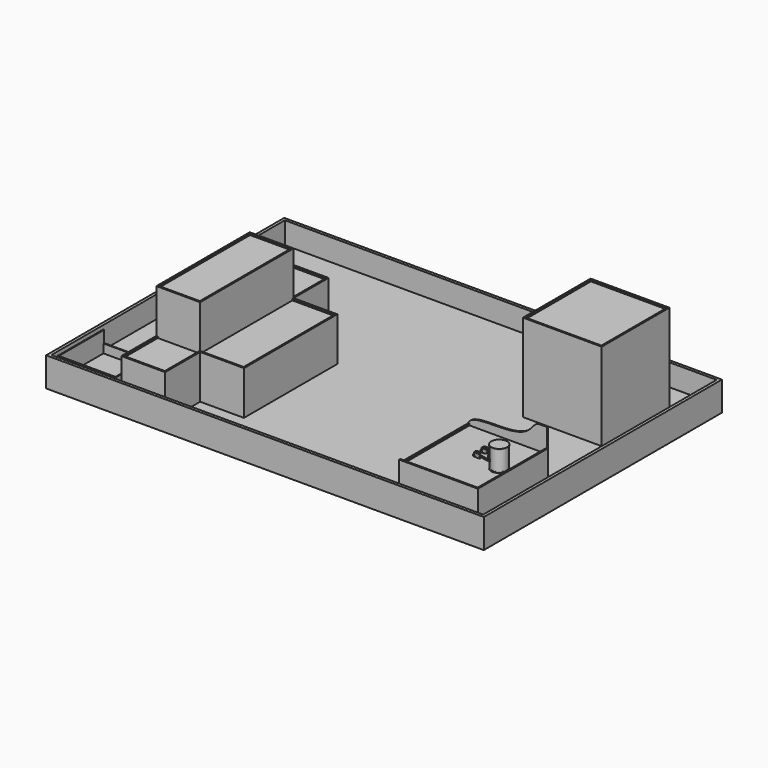
from build123d import *

# Parameters (mm, degrees)
F0_R      = 27.2
F1_DEPTH  = 2.83
F2_R      = 26.4
F3_DEPTH  = 67.36
F4_R      = 27.2
F5_DEPTH  = 2.83
F9_W      = 270
F9_H      = 300
F10_DEPTH = 72
F12_DEPTH = 15
F14_DEPTH = 5
F15_W     = 5
F15_H     = 290
F16_DEPTH = 5
F17_W     = 1500
F17_H     = 1020
F18_DEPTH = 25
F19_W     = 270
F19_H     = 290
F20_DEPTH = 300
F21_W     = 260
F21_H     = 280
F22_DEPTH = 5
F23_W     = 1500
F23_H     = 1020
F23_W_2   = 1480
F23_H_2   = 1000
F24_DEPTH = 75
F26_DEPTH = 150
F27_W     = 150
F27_H     = 400
F28_DEPTH = 150
F29_W     = 140
F29_H     = 390
F30_DEPTH = 5
F31_W     = 140
F31_H     = 145
F31_W_2   = 145
F31_H_2   = 390
F32_DEPTH = 5
F33_R     = 3
F34_DEPTH = 4
F35_R     = 3.99999
F35_2_R   = 3.99999
F36_R     = 3
F37_DEPTH = 8
F38_R     = 3
F39_DEPTH = 8
F40_R     = 3
F40_R_2   = 2.5
F41_DEPTH = 3
F42_R     = 3
F42_R_2   = 2.5
F43_DEPTH = 3
F45_DEPTH = 270.001
F46_W     = 200
F46_H     = 200
F46_W_2   = 194
F46_H_2   = 191
F47_DEPTH = 30
F49_DEPTH = 40
F50_R     = 2.7849277151
F50_R_2   = 2.6702247342
F50_R_3   = 2.7139155057
F50_R_4   = 2.7469543797
F51_DEPTH = 6


# Not quite as in the source:
# - a fillet or chamfer is up to 0.001 mm smaller than in the source, because OpenCascade refuses the exact size
# - a feature names something its author has since deleted; it is built from what else it names


with BuildPart() as f1:
    # F0 (on Top) → F1 (new body)
    with BuildSketch(Plane.XY):
        Circle(F0_R)
    extrude(amount=F1_DEPTH)

    # F2 (on face) → F3 (join)
    with BuildSketch(Plane.XY.offset(2.83)):
        Circle(F2_R)
    extrude(amount=F3_DEPTH)

    # F4 (on face) → F5 (join)
    with BuildSketch(Plane.XY.offset(70.19)):
        Circle(F4_R)
    extrude(amount=F5_DEPTH)


with BuildPart() as f10:
    # F9 (on Top) → F10 (new body)
    with BuildSketch(Plane.XY):
        with Locations((-87.8, 0)):
            Rectangle(F9_W, F9_H)
    extrude(amount=-F10_DEPTH)

    # F11 (on face) → F12 (join)
    with BuildSketch(Plane.XY):
        Polygon((-222.8, -145), (-222.8, -150), (47.2, -150), (47.2, 150), (42.2, 150), (42.2, -145), align=None)
    extrude(amount=F12_DEPTH)

    # F13 (on face) → F14 (join)
    with BuildSketch(Plane(origin=(0, 150, 0), x_dir=(-1, 0, 0), z_dir=(0, 1, 0))):
        with BuildLine():
            Line((-21.3134280931, 81.3575685024), (-47.2, 81.3575685024))
            Line((-47.2, 81.3575685024), (-47.2, -72))
            Line((-47.2, -72), (222.8, -72))
            Line((222.8, -72), (222.8, 0))
            add(Edge.make_bspline(
                [(-21.3134280931, 81.3575685024), (-6.3059147253, 81.3822787863), (12.9585432644, 38.1268753575), (103.6097013063, 23.6068887567), (223.0224295336, 30.7718731823), (222.8, 0)],
                knots=[0, 0, 0, 0, 0.2487100673, 0.6151112321, 1, 1, 1, 1], degree=3))
        make_face()
    extrude(amount=-F14_DEPTH)

    # F15 (on face) → F16 (join)
    with BuildSketch(Plane.XY):
        with Locations((-220.3, 0)):
            Rectangle(F15_W, F15_H)
    extrude(amount=F16_DEPTH)

    # F17 (on face) → F18 (join)
    with BuildSketch(Plane(origin=(0, 0, -72), x_dir=(1, 0, 0), z_dir=(0, 0, -1))):
        with Locations((-602.8, -260)):
            Rectangle(F17_W, F17_H)
    extrude(amount=F18_DEPTH)

    # F19 (on face) → F20 (join)
    with BuildSketch(Plane.XY.offset(-72)):
        with Locations((-87.8, 525)):
            Rectangle(F19_W, F19_H)
    extrude(amount=F20_DEPTH)

    # F21 (on face) → F22 (cut)
    with BuildSketch(Plane.XY.offset(228)):
        with Locations((-87.8, 525)):
            Rectangle(F21_W, F21_H)
    extrude(amount=-F22_DEPTH, mode=Mode.SUBTRACT)

    # F23 (on face) → F24 (join)
    with BuildSketch(Plane.XY.offset(-72)):
        with Locations((-602.8, 260)):
            Rectangle(F23_W, F23_H)
        with Locations((-602.8, 260)):
            Rectangle(F23_W_2, F23_H_2, mode=Mode.SUBTRACT)
    extrude(amount=F24_DEPTH)

    # F25 (on face) → F26 (join)
    with BuildSketch(Plane.XY.offset(-72)):
        Polygon((-952.8, 460), (-1102.8, 460), (-1102.8, -240), (-952.8, -240), (-952.8, -90), (-802.8, -90), (-802.8, 310), (-952.8, 310), align=None)
    extrude(amount=F26_DEPTH)

    # F27 (on face) → F28 (join)
    with BuildSketch(Plane.XY.offset(78)):
        with Locations((-1027.8, 110)):
            Rectangle(F27_W, F27_H)
    extrude(amount=F28_DEPTH)

    # F29 (on face) → F30 (cut)
    with BuildSketch(Plane.XY.offset(228)):
        with Locations((-1027.8, 110)):
            Rectangle(F29_W, F29_H)
    extrude(amount=-F30_DEPTH, mode=Mode.SUBTRACT)

    # F31 (on face) → F32 (cut)
    with BuildSketch(Plane.XY.offset(78)):
        with Locations((-1027.8, 382.5)):
            Rectangle(F31_W, F31_H)
        with Locations((-880.3, 110)):
            Rectangle(F31_W_2, F31_H_2)
        with Locations((-1027.8, -162.5)):
            Rectangle(F31_W, F31_H)
    extrude(amount=-F32_DEPTH, mode=Mode.SUBTRACT)

    # F46 (on face) → F47 (join)
    with BuildSketch(Plane.XY.offset(-72)):
        with Locations((-1232.8, -130)):
            Rectangle(F46_W, F46_H)
        with Locations((-1232.8, -128.5)):
            Rectangle(F46_W_2, F46_H_2, mode=Mode.SUBTRACT)
    extrude(amount=F47_DEPTH)

    # F48 (on face) → F49 (join)
    with BuildSketch(Plane.XY.offset(-42)):
        Polygon((-1329.8, -30), (-1332.8, -30), (-1332.8, -230), (-1329.8, -230), (-1135.8, -230), (-1132.8, -230), (-1132.8, -30), (-1135.8, -30), (-1135.8, -224), (-1329.8, -224), align=None)
    extrude(amount=F49_DEPTH)


with BuildPart() as f34:
    # F33 (on offset) → F34 (new body, symmetric)
    with BuildSketch(Plane.XY.offset(25)):
        with BuildLine():
            Line((-55, -12), (-74.5, -12))
            Line((-74.5, -12), (-74.5, -13))
            Line((-74.5, -13), (-65.6457513111, -13))
            ThreePointArc((-65.6457513111, -13), (-67, -16), (-65.6457513111, -19))
            Line((-65.6457513111, -19), (-74.5, -19))
            Line((-74.5, -19), (-74.5, -20))
            Line((-74.5, -20), (-55, -20))
            ThreePointArc((-55, -20), (-51, -16), (-55, -12))
        make_face()
        with Locations((-63, -16)):
            Circle(F33_R, mode=Mode.SUBTRACT)
        with Locations((-55, -16)):
            Circle(F33_R, mode=Mode.SUBTRACT)
    extrude(amount=F34_DEPTH, both=True)

    # F35 (radius 4 in the source; OpenCascade refuses exactly that, so slightly less here)
    f35_edges = [f34.edges().sort_by_distance(p)[0] for p in [
        (-74.5, -19.5, 29),
        (-74.5, -12.5, 29),
        (-74.5, -19.5, 21),
        (-74.5, -12.5, 21),
    ]]
    fillet(f35_edges, radius=F35_R)

    # F36 (on face) → F37 (join, through all)
    with BuildSketch(Plane.XZ.offset(20)):
        with Locations((-70.5, 25)):
            Circle(F36_R)
    extrude(amount=-F37_DEPTH)

    # F42 (on offset) → F43 (join, symmetric)
    with BuildSketch(Plane.XY.offset(25)):
        with Locations((-63, -16)):
            Circle(F42_R)
        with Locations((-63, -16)):
            Circle(F42_R_2, mode=Mode.SUBTRACT)
        with Locations((-55, -16)):
            Circle(F42_R)
        with Locations((-55, -16)):
            Circle(F42_R_2, mode=Mode.SUBTRACT)
    extrude(amount=F43_DEPTH, both=True)


with BuildPart() as f34b:
    # F33 (on offset) → F34, piece 2 (new body, symmetric)
    with BuildSketch(Plane.XY.offset(25)):
        with BuildLine():
            Line((-74.5, 13), (-74.5, 12))
            Line((-74.5, 12), (-55, 12))
            ThreePointArc((-55, 12), (-51, 16), (-55, 20))
            Line((-55, 20), (-74.5, 20))
            Line((-74.5, 20), (-74.5, 19))
            Line((-74.5, 19), (-65.6457513111, 19))
            ThreePointArc((-65.6457513111, 19), (-67, 16), (-65.6457513111, 13))
            Line((-65.6457513111, 13), (-74.5, 13))
        make_face()
        with Locations((-63, 16)):
            Circle(F33_R, mode=Mode.SUBTRACT)
        with Locations((-55, 16)):
            Circle(F33_R, mode=Mode.SUBTRACT)
    extrude(amount=F34_DEPTH, both=True)

    # F35#2 (radius 4 in the source; OpenCascade refuses exactly that, so slightly less here)
    f35_2_edges = [f34b.edges().sort_by_distance(p)[0] for p in [
        (-74.5, 12.5, 29),
        (-74.5, 19.5, 29),
        (-74.5, 19.5, 21),
        (-74.5, 12.5, 21),
    ]]
    fillet(f35_2_edges, radius=F35_2_R)

    # F38 (on face) → F39 (join, through all)
    with BuildSketch(Plane(origin=(0, 20, 0), x_dir=(-1, 0, 0), z_dir=(0, 1, 0))):
        with Locations((70.5, 25)):
            Circle(F38_R)
    extrude(amount=-F39_DEPTH)

    # F40 (on offset) → F41 (join, symmetric)
    with BuildSketch(Plane.XY.offset(25)):
        with Locations((-55, 16)):
            Circle(F40_R)
        with Locations((-55, 16)):
            Circle(F40_R_2, mode=Mode.SUBTRACT)
        with Locations((-63, 16)):
            Circle(F40_R)
        with Locations((-63, 16)):
            Circle(F40_R_2, mode=Mode.SUBTRACT)
    extrude(amount=F41_DEPTH, both=True)


with BuildPart() as f45_tool:
    # F44 (on face) → F45 (new body, through all)
    with BuildSketch(Plane(origin=(0, 20, 0), x_dir=(-1, 0, 0), z_dir=(0, 1, 0))):
        with BuildLine():
            Line((71.5, 26), (71.5, 27.2912878475))
            ThreePointArc((71.5, 27.2912878475), (70.5, 27.5), (69.5, 27.2912878475))
            Line((69.5, 27.2912878475), (69.5, 26))
            Line((69.5, 26), (68.2087121525, 26))
            ThreePointArc((68.2087121525, 26), (68, 25), (68.2087121525, 24))
            Line((68.2087121525, 24), (69.5, 24))
            Line((69.5, 24), (69.5, 22.7087121525))
            ThreePointArc((69.5, 22.7087121525), (70.5, 22.5), (71.5, 22.7087121525))
            Line((71.5, 22.7087121525), (71.5, 24))
            Line((71.5, 24), (72.7912878475, 24))
            ThreePointArc((72.7912878475, 24), (73, 25), (72.7912878475, 26))
            Line((72.7912878475, 26), (71.5, 26))
        make_face()
    extrude(amount=-F45_DEPTH)


with BuildPart() as f34_1:
    add(f34.part)

    # F45: cut by f45_tool
    add(f45_tool.part, mode=Mode.SUBTRACT)


with BuildPart() as f34b_1:
    add(f34b.part)

    # F45: cut by f45_tool
    add(f45_tool.part, mode=Mode.SUBTRACT)


with BuildPart() as f51:
    # F50 (on face) → F51 (new body)
    with BuildSketch(Plane.XY.offset(29)):
        with BuildLine():
            ThreePointArc((-7.5719285872, -28.1189057083), (-30.9613660003, -0.0256152683), (-6.4810490801, 27.1223650201))
            Line((-6.4810490801, 27.1223650201), (-19.0808027875, 27.1223650201))
            Line((-19.0808027875, 27.1223650201), (-53.2907301045, 23.6055955165))
            Line((-53.2907301045, 23.6055955165), (-66.5, 23.6055955165))
            ThreePointArc((-66.5, 23.6055955165), (-69.3284271247, 22.4340226413), (-70.5, 19.6055955165))
            Line((-70.5, 19.6055955165), (-70.5, 14.3255915258))
            ThreePointArc((-70.5, 14.3255915258), (-69.3284271247, 11.4971644011), (-66.5, 10.3255915258))
            Line((-66.5, 10.3255915258), (-45.6036029027, 10.3255915258))
            ThreePointArc((-45.6036029027, 10.3255915258), (-38.5325350909, 7.3966593377), (-35.6036029027, 0.3255915258))
            Line((-35.6036029027, 0.3255915258), (-35.6036029027, -0.0644301791))
            ThreePointArc((-35.6036029027, -0.0644301791), (-38.5325350909, -7.135497991), (-45.6036029027, -10.0644301791))
            Line((-45.6036029027, -10.0644301791), (-66.5, -10.0644301791))
            ThreePointArc((-66.5, -10.0644301791), (-69.3284271247, -11.2360030544), (-70.5, -14.0644301791))
            Line((-70.5, -14.0644301791), (-70.5, -17.4790090423))
            ThreePointArc((-70.5, -17.4790090423), (-69.3284271247, -20.307436167), (-66.5, -21.4790090423))
            Line((-66.5, -21.4790090423), (-53.2907301045, -21.4790090423))
            Line((-53.2907301045, -21.4790090423), (-19.0808027875, -28.2756832567))
            Line((-19.0808027875, -28.2756832567), (-7.5719285872, -28.1189057083))
        make_face()
        with Locations((-62.9321113229, -16.0951223224)):
            Circle(F50_R, mode=Mode.SUBTRACT)
        with Locations((-55, -16)):
            Circle(F50_R_2, mode=Mode.SUBTRACT)
        with Locations((-63, 16)):
            Circle(F50_R_3, mode=Mode.SUBTRACT)
        with Locations((-55, 16)):
            Circle(F50_R_4, mode=Mode.SUBTRACT)
    extrude(amount=F51_DEPTH)


solid = Compound([f1.part, f10.part, f34_1.part, f34b_1.part, f51.part])
